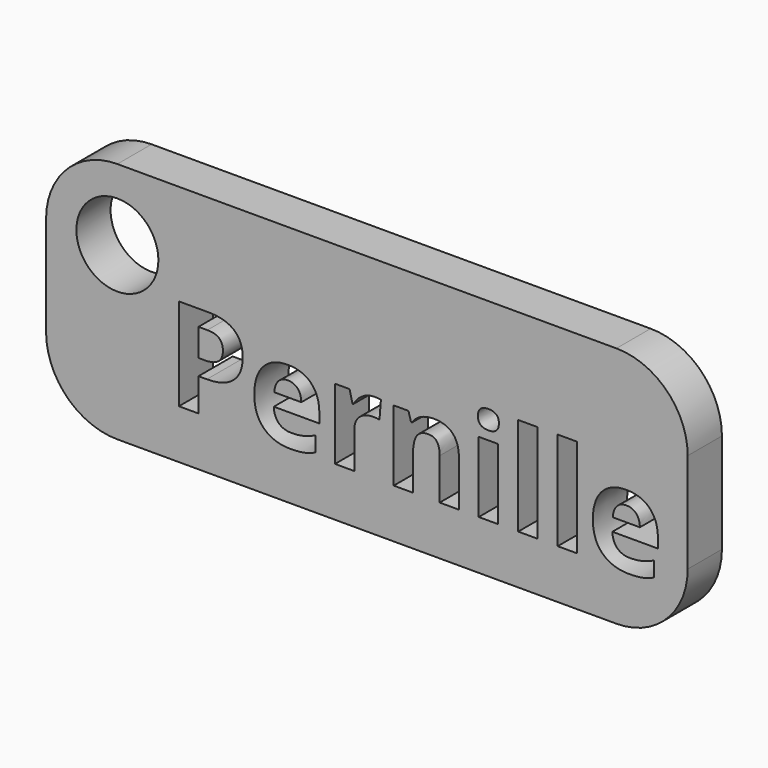
from build123d import *

# Parameters (mm, degrees)
F1_DEPTH     = 3
F2_R         = 2.8764797093
F3_DEPTH     = 3
F4_TEXT_SIZE = 9.0717641341
F5_DEPTH     = 3


# Not quite as in the source:
# - Text() gives the source's letters only with a copy of the font that has no kerning and outlines rounded to 1/6400 em; it was checked with that copy


with BuildPart() as f1:
    # F0 (on Front) → F1 (new body)
    with BuildSketch(Plane.XZ):
        with BuildLine():
            Line((27.1153831109, 2.6291993682), (-7.8846168891, 2.6291993682))
            ThreePointArc((-7.8846168891, 2.6291993682), (-11.420150795, 1.1647332741), (-12.8846168891, -2.3708006318))
            Line((-12.8846168891, -2.3708006318), (-12.8846168891, -9.3708006318))
            ThreePointArc((-12.8846168891, -9.3708006318), (-11.420150795, -12.9063345377), (-7.8846168891, -14.3708006318))
            Line((-7.8846168891, -14.3708006318), (27.1153831109, -14.3708006318))
            ThreePointArc((27.1153831109, -14.3708006318), (30.6509170169, -12.9063345377), (32.1153831109, -9.3708006318))
            Line((32.1153831109, -9.3708006318), (32.1153831109, -2.3708006318))
            ThreePointArc((32.1153831109, -2.3708006318), (30.6509170169, 1.1647332741), (27.1153831109, 2.6291993682))
        make_face()
    extrude(amount=F1_DEPTH)

    # F2 (on face) → F3 (cut)
    with BuildSketch(Plane.XZ.offset(3)):
        with Locations((-7.8846168891, -2.3708006318)):
            Circle(F2_R)
    extrude(amount=-F3_DEPTH, mode=Mode.SUBTRACT)

    # F4 (on face) → F5 (cut)
    with BuildSketch(Plane.XZ.offset(3)):
        with Locations((-4.3855497013, -10.9224757734)):
            Text('Pernille', F4_TEXT_SIZE, font='Open Sans', font_style=FontStyle.BOLD, text_align=(TextAlign.LEFT, TextAlign.BOTTOM))
    extrude(amount=-F5_DEPTH, mode=Mode.SUBTRACT)


solid = f1.part
